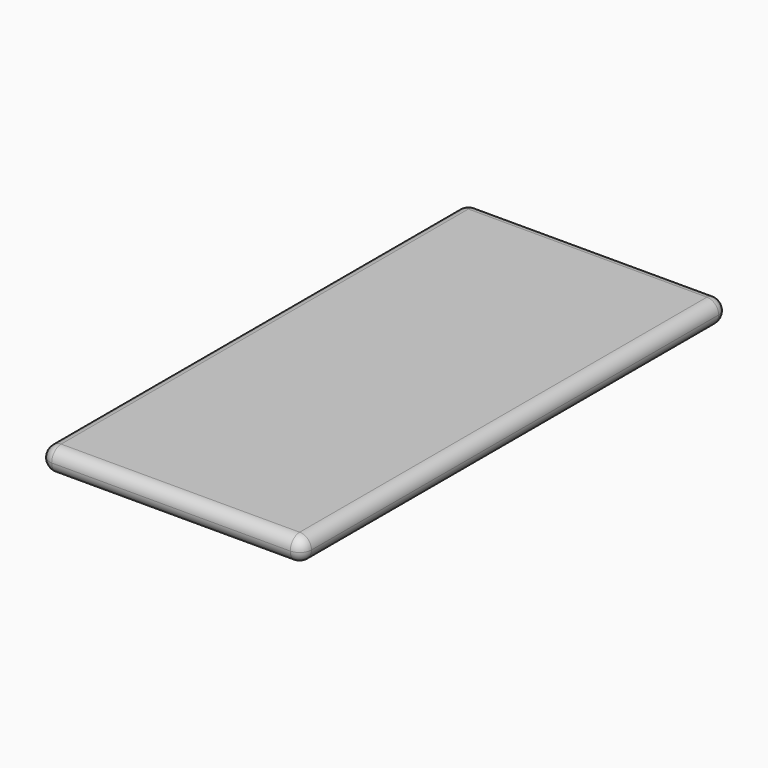
from build123d import *

# Parameters (mm, degrees)
F0_W     = 78
F0_H     = 158.5
F0_R     = 5.75
F0_R_2   = 0.75
F0_W_2   = 14
F0_H_2   = 1
F0_W_3   = 22
F0_H_3   = 12
F1_DEPTH = 7
F2_R     = 3.49999


# Not quite as in the source:
# - a fillet or chamfer is up to 0.001 mm smaller than in the source, because OpenCascade refuses the exact size


with BuildPart() as f1:
    # F0 (on Top) → F1 (new body)
    with BuildSketch(Plane.XY):
        Rectangle(F0_W, F0_H)
        with Locations((0, -69.5)):
            Circle(F0_R, mode=Mode.SUBTRACT)
        with Locations((-13.75, 69.75)):
            Circle(F0_R_2, mode=Mode.SUBTRACT)
        with Locations((0, 69.75)):
            Rectangle(F0_W_2, F0_H_2, mode=Mode.SUBTRACT)
        with Locations((22.5, 67.75)):
            Rectangle(F0_W_3, F0_H_3, mode=Mode.SUBTRACT)
        with Locations((0, -69.5)):
            Circle(F0_R)
        with Locations((22.5, 67.75)):
            Rectangle(F0_W_3, F0_H_3)
        with Locations((0, 69.75)):
            Rectangle(F0_W_2, F0_H_2)
        with Locations((-13.75, 69.75)):
            Circle(F0_R_2)
    extrude(amount=F1_DEPTH)

    # F2 (radius 3.5 in the source; OpenCascade refuses exactly that, so slightly less here)
    f2_edges = [f1.edges().sort_by_distance(p)[0] for p in [
        (39, 0, 7),
        (-39, 0, 7),
        (0, -79.25, 7),
        (0, 79.25, 7),
        (39, 0, 0),
        (0, -79.25, 0),
        (0, 79.25, 0),
        (-39, 0, 0),
        (-39, 79.25, 3.5),
        (39, 79.25, 3.5),
        (-39, -79.25, 3.5),
        (39, -79.25, 3.5),
    ]]
    fillet(f2_edges, radius=F2_R)


solid = f1.part
